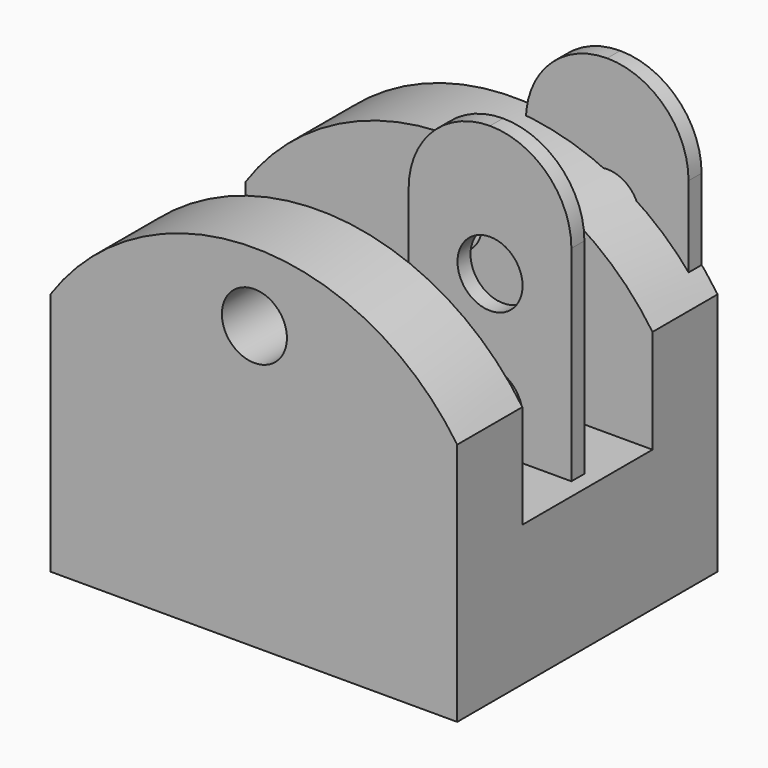
from build123d import *

# Parameters (mm, degrees)
F0_R     = 10.16
F1_DEPTH = 101.6
F2_W     = 50.8
F2_H     = 32.354841419
F2_H_2   = 44.4474281366
F3_DEPTH = 254
F4_R     = 10.16
F5_DEPTH = 50.8
F6_W     = 40.64
F6_H     = 34.1181978053
F6_H_2   = 66.04
F6_H_3   = 31.4270798117
F7_DEPTH = 76.2


with BuildPart() as f1:
    # F0 (on Front) → F1 (new body)
    with BuildSketch(Plane.XZ):
        with BuildLine():
            Line((-63.6832991838, 26.3976244633), (-63.6832991838, -49.8023755367))
            Line((-63.6832991838, -49.8023755367), (63.3167008162, -49.8023755367))
            Line((63.3167008162, -49.8023755367), (63.3167008162, 26.3976244633))
            ThreePointArc((63.3167008162, 26.3976244633), (-0.1832991838, 59.8891982699), (-63.6832991838, 26.3976244633))
        make_face()
        with Locations((0, 38.4011343122)):
            Circle(F0_R, mode=Mode.SUBTRACT)
    extrude(amount=F1_DEPTH)

    # F2 (on face) → F3 (cut)
    with BuildSketch(Plane(origin=(-63.6832991838, 0, 0), x_dir=(0, -1, 0), z_dir=(-1, 0, 0))):
        with Locations((50.8, 10.2202037538)):
            Rectangle(F2_W, F2_H)
        with Locations((50.8, 48.6213385316)):
            Rectangle(F2_W, F2_H_2)
    extrude(amount=-F3_DEPTH, mode=Mode.SUBTRACT)


with BuildPart() as f5:
    # F4 (on Front) → F5 (new body)
    with BuildSketch(Plane.XZ):
        with BuildLine():
            ThreePointArc((58.3152576901, 58.0664948159), (50.8757699322, 76.0270070581), (32.9152576901, 83.4664948159))
            ThreePointArc((32.9152576901, 83.4664948159), (14.954745448, 76.0270070581), (7.5152576901, 58.0664948159))
            Line((7.5152576901, 58.0664948159), (7.5152576901, 42.8264948159))
            Line((7.5152576901, 42.8264948159), (7.5152576901, -7.9735051841))
            ThreePointArc((7.5152576901, -7.9735051841), (32.9152576901, -33.3735051841), (58.3152576901, -7.9735051841))
            Line((58.3152576901, -7.9735051841), (58.3152576901, 42.8264948159))
            Line((58.3152576901, 42.8264948159), (58.3152576901, 58.0664948159))
        make_face()
        with Locations((32.9152576901, 7.2664948159)):
            Circle(F4_R, mode=Mode.SUBTRACT)
        with BuildLine():
            ThreePointArc((32.9152576901, 52.9864948159), (40.099462587, 50.0106997128), (43.0752576901, 42.8264948159))
            ThreePointArc((43.0752576901, 42.8264948159), (25.7310527932, 35.6422899191), (32.9152576901, 52.9864948159))
        make_face(mode=Mode.SUBTRACT)
    extrude(amount=F5_DEPTH)

    # F6 (on face) → F7 (cut)
    with BuildSketch(Plane.YZ.offset(58.3152576901)):
        with Locations((-25.4, 75.1255937186)):
            Rectangle(F6_W, F6_H)
        with Locations((-25.4, 25.0464948159)):
            Rectangle(F6_W, F6_H_2)
        with Locations((-25.4, -23.6870450899)):
            Rectangle(F6_W, F6_H_3)
    extrude(amount=-F7_DEPTH, mode=Mode.SUBTRACT)


solid = Compound([f1.part, f5.part])
